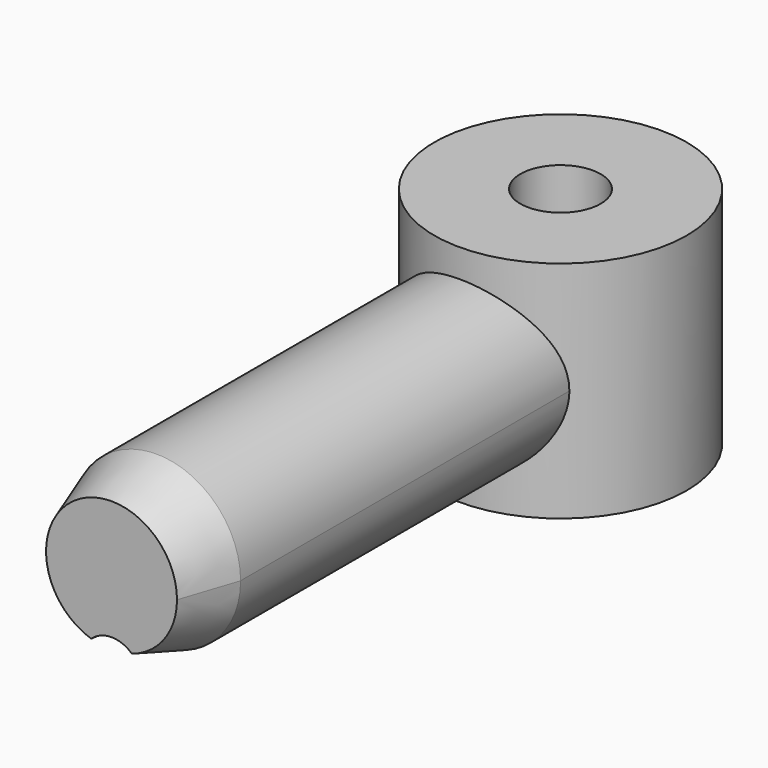
from build123d import *

# Parameters (mm, degrees)
F0_R          = 6.75
F0_R_2        = 2.15
F1_DEPTH      = 6
F1_DEPTH_BACK = 6
F3_START      = 5
F3_DEPTH      = 25
F4_SIZE2      = 3
F4_SIZE       = 1


with BuildPart() as f1:
    # F0 (on Top) → F1 (new body, two sides)
    with BuildSketch(Plane.XY) as f1_sk:
        Circle(F0_R)
        Circle(F0_R_2, mode=Mode.SUBTRACT)
    extrude(amount=F1_DEPTH)
    extrude(f1_sk.sketch, amount=-F1_DEPTH_BACK)

    # F2 (on Front) → F3 (join)
    with BuildSketch(Plane.XZ.offset(F3_START)):
        with BuildLine():
            ThreePointArc((1.5745130543, -4.2155555556), (3.6969790873, -2.5656082374), (4.5, 0))
            ThreePointArc((4.5, 0), (-2.5656082374, 3.6969790873), (-1.5745130543, -4.2155555556))
            ThreePointArc((-1.5745130543, -4.2155555556), (0, -2.9), (1.5745130543, -4.2155555556))
        make_face()
    extrude(amount=F3_DEPTH)

    # F4
    f4_edges = [f1.edges().sort_by_distance(p)[0] for p in [
        (0, -30, 4.5),
    ]]
    f4_side = f1.faces().sort_by_distance((0, -30, 0.234076))[0]
    chamfer(f4_edges, length=F4_SIZE, length2=F4_SIZE2, reference=f4_side)


solid = f1.part
